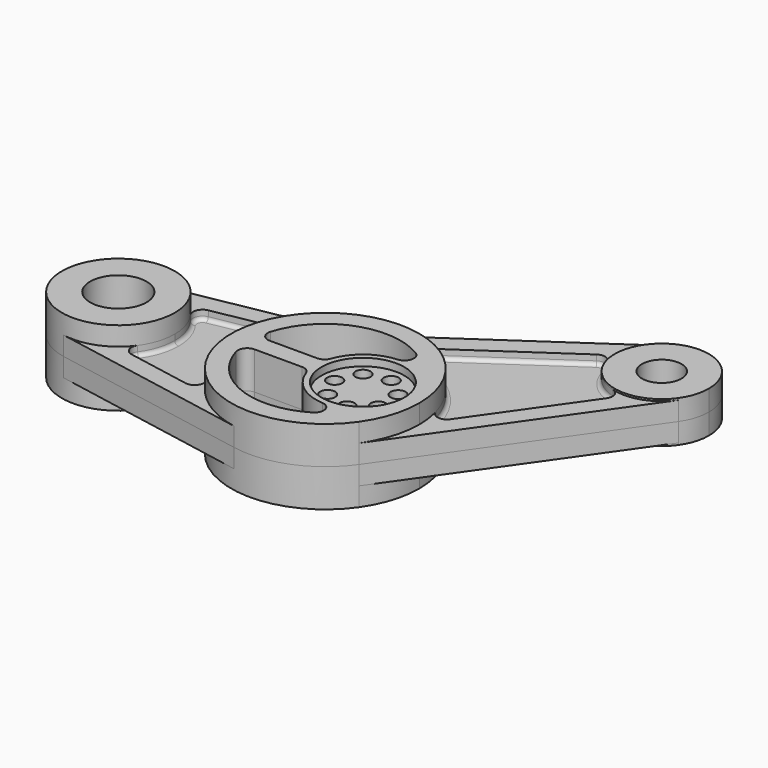
from build123d import *

# Parameters (mm, degrees)
F0_R     = 15
F1_DEPTH = 20
F0_R_2   = 22
F2_DEPTH = 20
F0_R_3   = 4
F3_DEPTH = 16
F0_R_4   = 10.5
F4_DEPTH = 11
F5_DEPTH = 10
F7_DEPTH = 5
F8_R     = 2


# Not quite as in the source:
# - a feature names something its author has since deleted; it is built from what else it names


with BuildPart() as f1:
    # F0 (on Top) → F1 (new body)
    with BuildSketch(Plane.XY):
        with BuildLine():
            ThreePointArc((-135.4545454545, -29.4999649811), (-110.811935528, -23.0611834436), (-100, 0))
            ThreePointArc((-100, 0), (-110.811935528, 23.0611834436), (-135.4545454545, 29.4999649811))
            ThreePointArc((-135.4545454545, 29.4999649811), (-160, 0), (-135.4545454545, -29.4999649811))
        make_face()
        with Locations((-130, 0)):
            Circle(F0_R, mode=Mode.SUBTRACT)
    extrude(amount=F1_DEPTH)



with BuildPart() as f2:
    # F0 (on Top) → F2 (new body)
    with BuildSketch(Plane.XY):
        with BuildLine():
            ThreePointArc((30, 0), (-51.9801074533, 38.4353057393), (-29.0909090909, -49.1666083018))
            ThreePointArc((-29.0909090909, -49.1666083018), (-1.0982935918, -46.2895830059), (20.9072911046, -28.7505397251))
            ThreePointArc((20.9072911046, -28.7505397251), (27.6726575472, -15.0770594741), (30, 0))
        make_face()
        with BuildLine():
            ThreePointArc((0.7142857143, -34.2186844772), (-34.4030729021, -37.3169062353), (-58.3325939, -11.4285714286))
            ThreePointArc((-58.3325939, -11.4285714286), (-57.5499382912, -7.0119284767), (-53.5410196625, -5))
            Line((-53.5410196625, -5), (-28.2842712475, -5))
            ThreePointArc((-28.2842712475, -5), (-25.3975199015, -5.9175170954), (-23.5702260396, -8.3333333333))
            ThreePointArc((-23.5702260396, -8.3333333333), (-15.0649003322, -19.9511598154), (-1.5625, -24.9511240979))
            ThreePointArc((-1.5625, -24.9511240979), (2.9806162254, -28.7484570232), (0.7142857143, -34.2186844772))
        make_face(mode=Mode.SUBTRACT)
        with BuildLine():
            Line((-28.2842712475, 5), (-53.5410196625, 5))
            ThreePointArc((-53.5410196625, 5), (-57.5499382912, 7.0119284767), (-58.3325939, 11.4285714286))
            ThreePointArc((-58.3325939, 11.4285714286), (-34.4030729021, 37.3169062353), (0.7142857143, 34.2186844772))
            ThreePointArc((0.7142857143, 34.2186844772), (2.9806162254, 28.7484570232), (-1.5625, 24.9511240979))
            ThreePointArc((-1.5625, 24.9511240979), (-15.0649003322, 19.9511598154), (-23.5702260396, 8.3333333333))
            ThreePointArc((-23.5702260396, 8.3333333333), (-25.3975199015, 5.9175170954), (-28.2842712475, 5))
        make_face(mode=Mode.SUBTRACT)
        Circle(F0_R_2, mode=Mode.SUBTRACT)
    extrude(amount=F2_DEPTH)

    # F0 (on Top) → F3 (join)
    with BuildSketch(Plane.XY):
        Circle(F0_R_2)
        with Locations((3.2465942091, -14.6444401068)):
            Circle(F0_R_3, mode=Mode.SUBTRACT)
        with Locations((-9.4398058657, -11.6571894219)):
            Circle(F0_R_3, mode=Mode.SUBTRACT)
        with Locations((-15, 0)):
            Circle(F0_R_3, mode=Mode.SUBTRACT)
        with Locations((-9.3377195496, 11.7391223528)):
            Circle(F0_R_3, mode=Mode.SUBTRACT)
        with Locations((3.3742658152, 14.6155509718)):
            Circle(F0_R_3, mode=Mode.SUBTRACT)
        with Locations((13.4819106945, -6.5755672018)):
            Circle(F0_R_3, mode=Mode.SUBTRACT)
        with Locations((13.5387792652, 6.4576664521)):
            Circle(F0_R_3, mode=Mode.SUBTRACT)
    extrude(amount=F3_DEPTH)


with BuildPart() as f4:
    # F0 (on Top) → F4 (new body)
    with BuildSketch(Plane.XY):
        with BuildLine():
            ThreePointArc((104.9236896633, 98.697537105), (91.5847091217, 120.8113478393), (65.8020396479, 119.3271032867))
            ThreePointArc((65.8020396479, 119.3271032867), (62.1372291248, 81.1293322591), (100.3773352156, 84.3222672425))
            ThreePointArc((100.3773352156, 84.3222672425), (103.7600184369, 91.159007368), (104.9236896633, 98.697537105))
        make_face()
        with Locations((79.9236896633, 98.697537105)):
            Circle(F0_R_4, mode=Mode.SUBTRACT)
    extrude(amount=F4_DEPTH)


with BuildPart() as f1_1:
    add(f1.part)

    add(f2.part)  # F5 merges F2

    add(f4.part)  # F5 merges F4
    # F0 (on Top) → F5 (join)
    with BuildSketch(Plane.XY):
        with BuildLine():
            ThreePointArc((-135.4545454545, 29.4999649811), (-110.811935528, 23.0611834436), (-100, 0))
            ThreePointArc((-100, 0), (-110.811935528, -23.0611834436), (-135.4545454545, -29.4999649811))
            Line((-135.4545454545, -29.4999649811), (-29.0909090909, -49.1666083018))
            ThreePointArc((-29.0909090909, -49.1666083018), (-51.9801074533, 38.4353057393), (30, 0))
            ThreePointArc((30, 0), (27.6726575472, -15.0770594741), (20.9072911046, -28.7505397251))
            Line((20.9072911046, -28.7505397251), (100.3773352156, 84.3222672425))
            ThreePointArc((100.3773352156, 84.3222672425), (62.1372291248, 81.1293322591), (65.8020396479, 119.3271032867))
            Line((65.8020396479, 119.3271032867), (-37.4072076356, 48.6768115811))
            ThreePointArc((-37.4072076356, 48.6768115811), (-39.6061075981, 47.487193189), (-42.0037814612, 46.7790173559))
            Line((-42.0037814612, 46.7790173559), (-135.4545454545, 29.4999649811))
        make_face()
    extrude(amount=F5_DEPTH)

    # F6 (on face) → F7 (cut)
    with BuildSketch(Plane.XY.offset(10)):
        with BuildLine():
            ThreePointArc((-100, 0), (-101.4564046173, -9.233805425), (-105.6842108418, -17.5710670597))
            ThreePointArc((-105.6842108418, -17.5710670597), (-106.2728456659, -22.3593219456), (-102.5406702246, -25.4162390665))
            Line((-102.5406702246, -25.4162390665), (-68.9919778385, -31.619394483))
            ThreePointArc((-68.9919778385, -31.619394483), (-64.0232375423, -29.621508542), (-63.7117153904, -24.2752124117))
            ThreePointArc((-63.7117153904, -24.2752124117), (-70, 0), (-63.7117153904, 24.2752124117))
            ThreePointArc((-63.7117153904, 24.2752124117), (-64.0232375423, 29.621508542), (-68.9919778385, 31.619394483))
            Line((-68.9919778385, 31.619394483), (-102.5406702246, 25.4162390665))
            ThreePointArc((-102.5406702246, 25.4162390665), (-106.2728456659, 22.3593219456), (-105.6842108418, 17.5710670597))
            ThreePointArc((-105.6842108418, 17.5710670597), (-101.4564046173, 9.233805425), (-100, 0))
        make_face()
        with BuildLine():
            ThreePointArc((-7.5851052887, 56.9725406605), (-9.6971025879, 52.0512201291), (-6.1461593506, 48.0423885674))
            ThreePointArc((-6.1461593506, 48.0423885674), (15.5729210771, 35.136409692), (28.2097688146, 13.2596452005))
            ThreePointArc((28.2097688146, 13.2596452005), (32.1744542827, 9.6594788843), (37.1214748065, 11.710555748))
            Line((37.1214748065, 11.710555748), (75.9321157128, 66.9317168355))
            ThreePointArc((75.9321157128, 66.9317168355), (76.550641894, 71.4869239552), (73.1884371125, 74.6218985242))
            ThreePointArc((73.1884371125, 74.6218985242), (62.1372291248, 81.1293322591), (55.7667314716, 92.260039849))
            ThreePointArc((55.7667314716, 92.260039849), (52.6735061963, 95.6606933064), (48.1110098301, 95.0984536341))
            Line((48.1110098301, 95.0984536341), (-7.5851052887, 56.9725406605))
        make_face()
    extrude(amount=-F7_DEPTH, mode=Mode.SUBTRACT)

    # F8
    f8_edges = [f1_1.edges().sort_by_distance(p)[0] for p in [
        (-85.766324, 28.517817, 5),
        (-100, 0, 5),
        (20.262952, 76.035497, 5),
        (62.137229, 81.129332, 5),
        (56.526795, 39.321136, 5),
        (-70, 0, 5),
        (-85.766324, -28.517817, 5),
    ]]
    fillet(f8_edges, radius=F8_R)

    # F9: F1 across plane


with BuildPart() as f1_2:
    add(f1_1.part)
    add(f1_1.part.mirror(Plane.XY))


solid = f1_2.part
